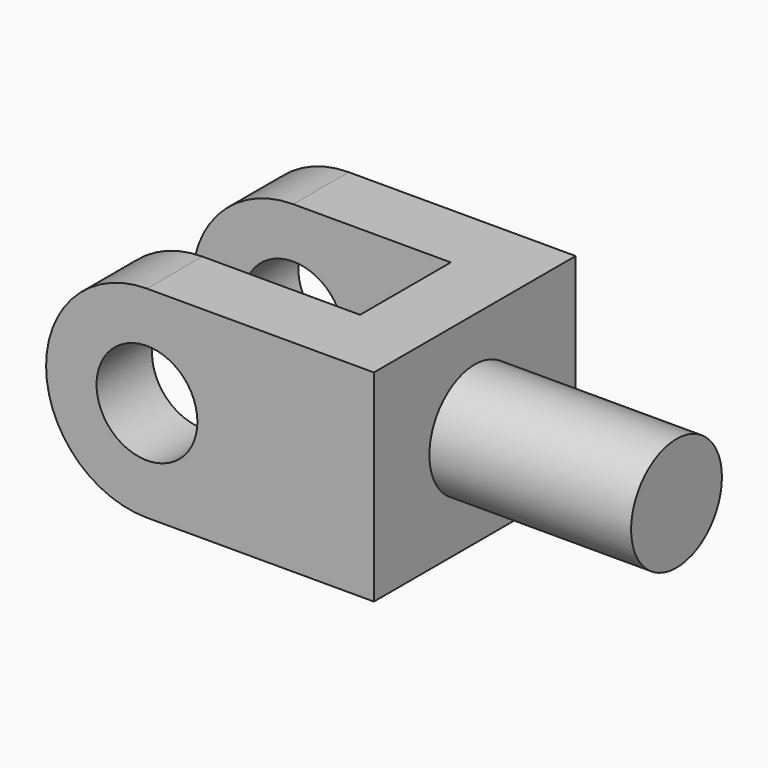
from build123d import *

# Parameters (mm, degrees)
F0_W     = 812.8
F0_H     = 457.2
F1_DEPTH = 812.8
F3_DEPTH = 812.8
F4_R     = 203.2
F5_DEPTH = 1016.001
F6_R     = 406.4
F7_R     = 406.39999
F8_R     = 406.4
F9_R     = 406.39999


# Not quite as in the source:
# - a fillet or chamfer is up to 0.001 mm smaller than in the source, because OpenCascade refuses the exact size


with BuildPart() as f1:
    # F0 (on Top) → F1 (new body)
    with BuildSketch(Plane.XY):
        Polygon((0, 279.4), (0, 0), (1320.8, 0), (1320.8, 279.4), (1320.8, 736.6), (1320.8, 1016), (0, 1016), (0, 736.6), (1041.4, 736.6), (1041.4, 279.4), align=None)
        with Locations((1727.2, 508)):
            Rectangle(F0_W, F0_H)
    extrude(amount=F1_DEPTH)

    # F2 (on face) → F3 (cut)
    with BuildSketch(Plane.YZ.offset(2133.6)):
        with BuildLine():
            ThreePointArc((279.4, 406.4), (508, 635), (736.6, 406.4))
            Line((736.6, 406.4), (736.6, 812.8))
            Line((736.6, 812.8), (279.4, 812.8))
            Line((279.4, 812.8), (279.4, 406.4))
        make_face()
        with BuildLine():
            Line((736.6, 0), (736.6, 406.4))
            ThreePointArc((736.6, 406.4), (508, 177.8), (279.4, 406.4))
            Line((279.4, 406.4), (279.4, 0))
            Line((279.4, 0), (736.6, 0))
        make_face()
    extrude(amount=-F3_DEPTH, mode=Mode.SUBTRACT)

    # F4 (on face) → F5 (cut, through all)
    with BuildSketch(Plane.XZ):
        with Locations((406.4, 406.4)):
            Circle(F4_R)
    extrude(amount=-F5_DEPTH, mode=Mode.SUBTRACT)

    # F6
    f6_edges = [f1.edges().sort_by_distance(p)[0] for p in [
        (0, 876.3, 812.8),
    ]]
    fillet(f6_edges, radius=F6_R)

    # F7 (radius 406.4 in the source; OpenCascade refuses exactly that, so slightly less here)
    f7_edges = [f1.edges().sort_by_distance(p)[0] for p in [
        (0, 876.3, 0),
    ]]
    fillet(f7_edges, radius=F7_R)

    # F8
    f8_edges = [f1.edges().sort_by_distance(p)[0] for p in [
        (0, 139.7, 0),
    ]]
    fillet(f8_edges, radius=F8_R)

    # F9 (radius 406.4 in the source; OpenCascade refuses exactly that, so slightly less here)
    f9_edges = [f1.edges().sort_by_distance(p)[0] for p in [
        (0, 139.7, 812.8),
    ]]
    fillet(f9_edges, radius=F9_R)


solid = f1.part
